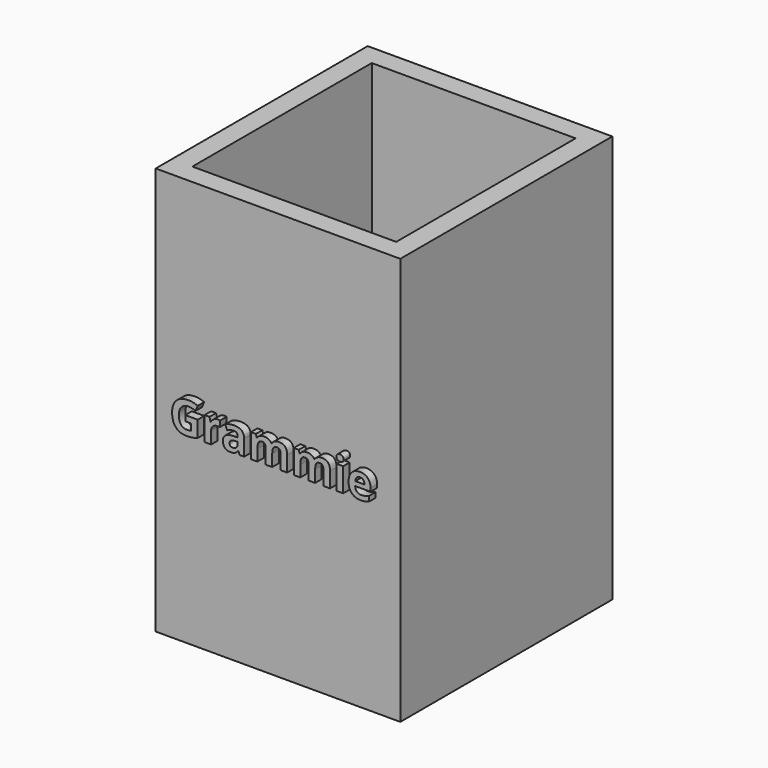
from build123d import *

# Parameters (mm, degrees)
F0_W         = 76.2
F0_H         = 127
F1_DEPTH     = 82.55
F2_W         = 63.5
F2_H         = 69.85
F3_DEPTH     = 120.65
F4_TEXT_SIZE = 13.61565264
F5_DEPTH     = 2.54


# Not quite as in the source:
# - Text() gives the source's letters only with a copy of the font that has no kerning and outlines rounded to 1/6400 em; it was checked with that copy


with BuildPart() as f1:
    # F0 (on Front) → F1 (new body)
    with BuildSketch(Plane.XZ):
        with Locations((-3.6884043366, -5.446185802)):
            Rectangle(F0_W, F0_H)
    extrude(amount=F1_DEPTH)

    # F2 (on face) → F3 (cut)
    with BuildSketch(Plane.XY.offset(58.053814198)):
        with Locations((-3.6884043366, -41.275)):
            Rectangle(F2_W, F2_H)
    extrude(amount=-F3_DEPTH, mode=Mode.SUBTRACT)

    # F4 (on face) → F5 (join)
    with BuildSketch(Plane.XZ.offset(82.55)):
        with Locations((-35.4384043366, -10.3472557028)):
            Text('Grammie', F4_TEXT_SIZE, font='Open Sans', font_style=FontStyle.BOLD, text_align=(TextAlign.LEFT, TextAlign.BOTTOM))
    extrude(amount=F5_DEPTH)


solid = f1.part
